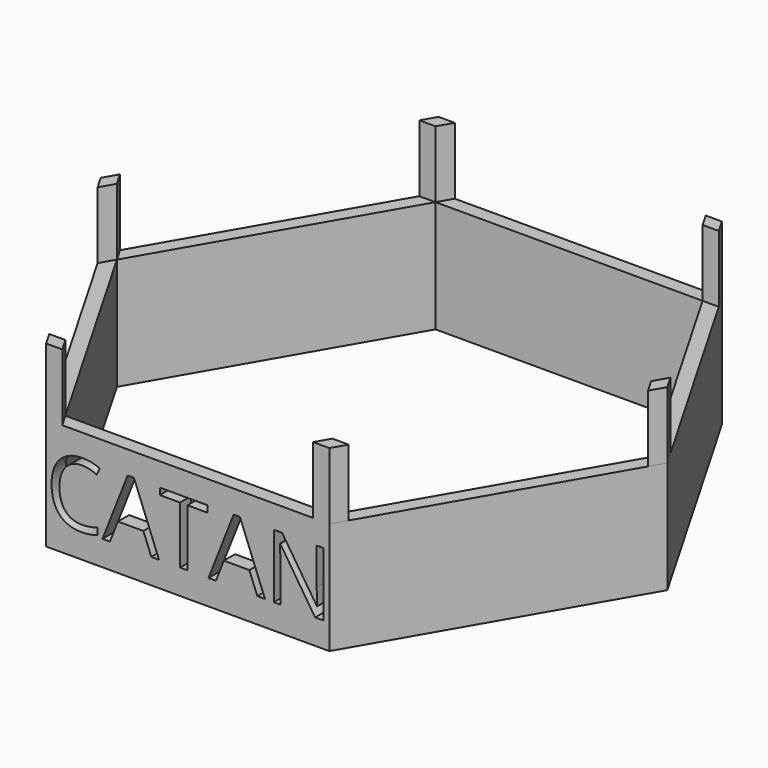
from build123d import *

# Parameters (mm, degrees)
F1_DEPTH     = 25
F3_DEPTH     = 14.9
F4_TEXT_SIZE = 19.9438413958
F5_DEPTH     = 25


# Not quite as in the source:
# - Text() gives the source's letters only with a copy of the font that has no kerning and outlines rounded to 1/6400 em; it was checked with that copy


with BuildPart() as f1:
    # F0 (on Top) → F1 (new body)
    with BuildSketch(Plane.XY):
        Polygon((31.6156629501, 54.7599345446), (-31.6156629501, 54.7599345446), (-63.2313259002, 0), (-31.6156629501, -54.7599345446), (31.6156629501, -54.7599345446), (63.2313259002, 0), align=None)
        Polygon((-59.6181110873, 0), (-29.8090555437, 51.6307987273), (29.8090555437, 51.6307987273), (59.6181110873, 0), (29.8090555437, -51.6307987273), (-29.8090555437, -51.6307987273), align=None, mode=Mode.SUBTRACT)
    extrude(amount=F1_DEPTH)

    # F2 (on face) → F3 (join)
    with BuildSketch(Plane.XY.offset(25)):
        Polygon((-33.4222703566, 51.6307987273), (-29.8090555437, 51.6307987273), (-28.0024481372, 54.7599345446), (-31.6156629501, 54.7599345446), align=None)
        Polygon((28.0024481372, 54.7599345446), (29.8090555437, 51.6307987273), (33.4222703566, 51.6307987273), (31.6156629501, 54.7599345446), align=None)
        Polygon((-61.4247184938, -3.1291358173), (-59.6181110873, 0), (-61.4247184938, 3.1291358173), (-63.2313259002, 0), align=None)
        Polygon((61.4247184938, 3.1291358173), (59.6181110873, 0), (61.4247184938, -3.1291358173), (63.2313259002, 0), align=None)
        Polygon((-28.0024481372, -54.7599345446), (-29.8090555437, -51.6307987273), (-33.4222703566, -51.6307987273), (-31.6156629501, -54.7599345446), align=None)
        Polygon((33.4222703566, -51.6307987273), (29.8090555437, -51.6307987273), (28.0024481372, -54.7599345446), (31.6156629501, -54.7599345446), align=None)
    extrude(amount=F3_DEPTH)

    # F4 (on face) → F5 (cut)
    with BuildSketch(Plane.XZ.offset(54.7599345446)):
        with Locations((-31.6156629501, 5.5904341951)):
            Text('CATAN', F4_TEXT_SIZE, font='Open Sans', text_align=(TextAlign.LEFT, TextAlign.BOTTOM))
        with BuildLine():
            Line((-15.0186474386, 11.6078650912), (-10.4128665662, 11.6078650912))
            Line((-10.4128665662, 11.6078650912), (-12.0706983823, 16.02044))
            add(Edge.make_bspline(
                [(-12.0706983823, 16.02044), (-12.3916695797, 16.8587045837), (-12.7313381285, 18.0740324187)],
                knots=[0, 0, 0, 1, 1, 1], degree=2))
            add(Edge.make_bspline(
                [(-12.7313381285, 18.0740324187), (-12.9463576685, 17.1391648533), (-13.3452344965, 16.02044)],
                knots=[0, 0, 0, 1, 1, 1], degree=2))
            Line((-13.3452344965, 16.02044), (-15.0186474386, 11.6078650912))
        make_face()
        with BuildLine():
            Line((8.6366181919, 11.6078650912), (13.2423990643, 11.6078650912))
            Line((13.2423990643, 11.6078650912), (11.5845672482, 16.02044))
            add(Edge.make_bspline(
                [(11.5845672482, 16.02044), (11.2635960508, 16.8587045837), (10.923927502, 18.0740324187)],
                knots=[0, 0, 0, 1, 1, 1], degree=2))
            add(Edge.make_bspline(
                [(10.923927502, 18.0740324187), (10.708907962, 17.1391648533), (10.310031134, 16.02044)],
                knots=[0, 0, 0, 1, 1, 1], degree=2))
            Line((10.310031134, 16.02044), (8.6366181919, 11.6078650912))
        make_face()
    extrude(amount=-F5_DEPTH, mode=Mode.SUBTRACT)


solid = f1.part
